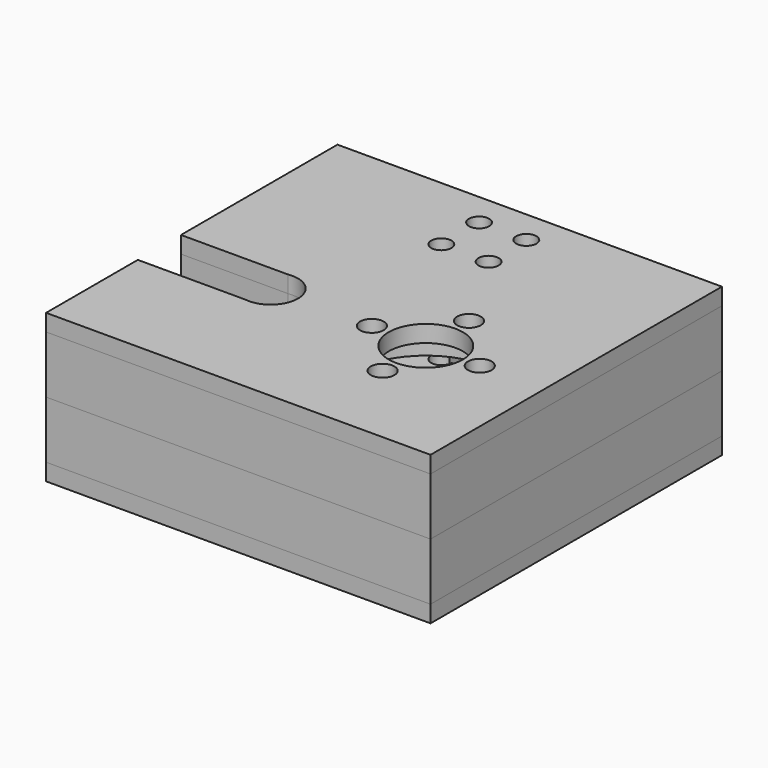
from build123d import *
from build123d import SkipClean  # not in build123d's __all__

# Parameters (mm, degrees)
F0_R     = 11
F0_W     = 51
F0_H     = 3
F1_DEPTH = 4.5
F2_DEPTH = 4
F3_R     = 1.75
F3_R_2   = 5.5
F3_R_3   = 1.5
F4_DEPTH = 2.5


with BuildPart() as f1:
    # F0 (on Top) → F1 (new body)
    with BuildSketch(Plane.XY):
        with BuildLine():
            Line((-14.5, 22.5), (-14.5, 26))
            Line((-14.5, 26), (-36.5, 26))
            Line((-36.5, 26), (-36.5, 4))
            Line((-36.5, 4), (-23.634428877, 4))
            ThreePointArc((-23.634428877, 4), (-20.3700700534, 3.0799299466), (-18.95, 0))
            ThreePointArc((-18.95, 0), (-20.3700700534, -3.0799299466), (-23.634428877, -4))
            Line((-23.634428877, -4), (-36.5, -4))
            Line((-36.5, -4), (-36.5, -18))
            Line((-36.5, -18), (14.5, -18))
            Line((14.5, -18), (14.5, 26))
            Line((14.5, 26), (-7.5, 26))
            Line((-7.5, 26), (-7.5, 22.5))
            ThreePointArc((-7.5, 22.5), (-6.4393398282, 22.0606601718), (-6, 21))
            ThreePointArc((-6, 21), (-7.5, 19.5), (-9, 21))
            Line((-9, 21), (-13, 21))
            ThreePointArc((-13, 21), (-15.5606601718, 19.9393398282), (-14.5, 22.5))
        make_face()
        Circle(F0_R, mode=Mode.SUBTRACT)
        with BuildLine():
            ThreePointArc((-14.5, 26.5), (-15.5606601718, 29.0606601718), (-13, 28))
            Line((-13, 28), (-9, 28))
            ThreePointArc((-9, 28), (-7.5, 29.5), (-6, 28))
            ThreePointArc((-6, 28), (-6.4393398282, 26.9393398282), (-7.5, 26.5))
            Line((-7.5, 26.5), (-7.5, 26))
            Line((-7.5, 26), (14.5, 26))
            Line((14.5, 26), (14.5, 33))
            Line((14.5, 33), (-36.5, 33))
            Line((-36.5, 33), (-36.5, 26))
            Line((-36.5, 26), (-14.5, 26))
            Line((-14.5, 26), (-14.5, 26.5))
        make_face()
        with Locations((-11, -19.5)):
            Rectangle(F0_W, F0_H)
        Polygon((14.5, 33), (14.5, 26), (14.5, -18), (14.5, -21), (17.5, -21), (17.5, 33), align=None)
        Polygon((-36.5, 4), (-36.5, 26), (-36.5, 33), (-39.5, 33), (-39.5, 4), align=None)
        Polygon((-36.5, -18), (-36.5, -4), (-39.5, -4), (-39.5, -21), (-36.5, -21), align=None)
    extrude(amount=F1_DEPTH)

    # F0 (on Top) → F2 (join)
    with BuildSketch(Plane.XY):
        Polygon((14.5, 33), (14.5, 26), (14.5, -18), (14.5, -21), (17.5, -21), (17.5, 33), align=None)
        with BuildLine():
            ThreePointArc((-14.5, 26.5), (-15.5606601718, 29.0606601718), (-13, 28))
            Line((-13, 28), (-9, 28))
            ThreePointArc((-9, 28), (-7.5, 29.5), (-6, 28))
            ThreePointArc((-6, 28), (-6.4393398282, 26.9393398282), (-7.5, 26.5))
            Line((-7.5, 26.5), (-7.5, 26))
            Line((-7.5, 26), (14.5, 26))
            Line((14.5, 26), (14.5, 33))
            Line((14.5, 33), (-36.5, 33))
            Line((-36.5, 33), (-36.5, 26))
            Line((-36.5, 26), (-14.5, 26))
            Line((-14.5, 26), (-14.5, 26.5))
        make_face()
        with Locations((-11, -19.5)):
            Rectangle(F0_W, F0_H)
        Polygon((-36.5, 4), (-36.5, 26), (-36.5, 33), (-39.5, 33), (-39.5, 4), align=None)
        Polygon((-36.5, -18), (-36.5, -4), (-39.5, -4), (-39.5, -21), (-36.5, -21), align=None)
    extrude(amount=-F2_DEPTH)

    # F3 (on face) → F4 (join)
    with BuildSketch(Plane.XY.offset(4.5)):
        with BuildLine():
            Line((-39.5, -4), (-39.5, -21))
            Line((-39.5, -21), (17.5, -21))
            Line((17.5, -21), (17.5, 33))
            Line((17.5, 33), (-39.5, 33))
            Line((-39.5, 33), (-39.5, 4))
            Line((-39.5, 4), (-23.634428877, 4))
            ThreePointArc((-23.634428877, 4), (-18.95, 0), (-23.634428877, -4))
            Line((-23.634428877, -4), (-39.5, -4))
        make_face()
        with Locations((0, -8)):
            Circle(F3_R, mode=Mode.SUBTRACT)
        with Locations((-8, 0)):
            Circle(F3_R, mode=Mode.SUBTRACT)
        Circle(F3_R_2, mode=Mode.SUBTRACT)
        with Locations((8, 0)):
            Circle(F3_R, mode=Mode.SUBTRACT)
        with Locations((-14.5, 21)):
            Circle(F3_R_3, mode=Mode.SUBTRACT)
        with Locations((-14.5, 28)):
            Circle(F3_R_3, mode=Mode.SUBTRACT)
        with Locations((0, 8)):
            Circle(F3_R, mode=Mode.SUBTRACT)
        with Locations((-7.5, 21)):
            Circle(F3_R_3, mode=Mode.SUBTRACT)
        with Locations((-7.5, 28)):
            Circle(F3_R_3, mode=Mode.SUBTRACT)
    with SkipClean():  # cleaning this boolean's faces spoils the solid; the shape is the same uncleaned
        extrude(amount=F4_DEPTH)


with BuildPart() as f5_1:
    # F5: instance of F1
    add(f1.part.mirror(Plane(origin=(-10.174939684, 11.2234552635, -4), x_dir=(1, 0, 0), z_dir=(0, 0, -1))), clean=False)


solid = Compound([f1.part, f5_1.part])
